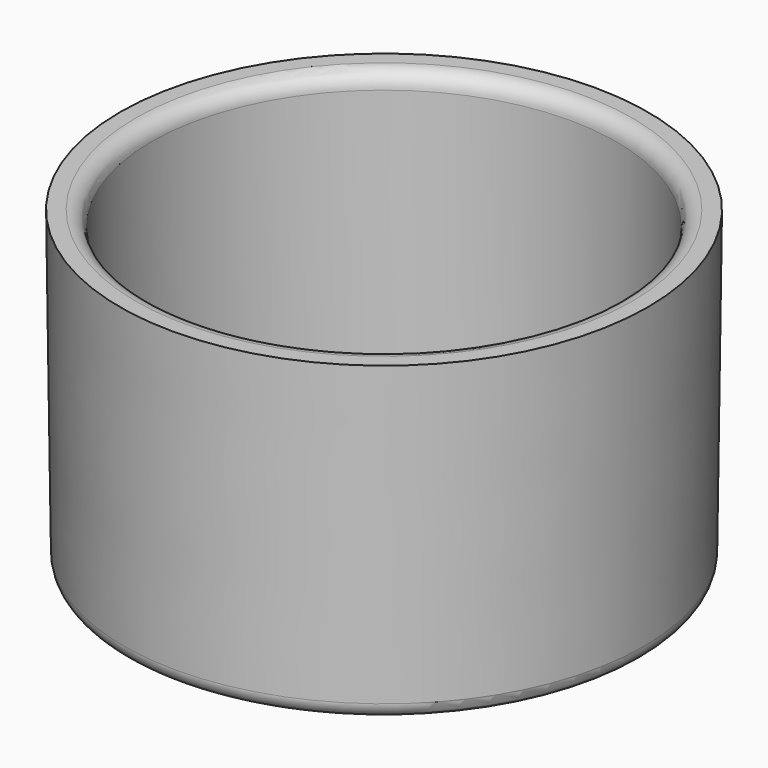
from build123d import *

# Parameters (mm, degrees)
F0_W     = 4
F0_H     = 40
F3_SIZE2 = 39.99999
F3_SIZE  = 0.49999
F4_R     = 2


# Not quite as in the source:
# - a fillet or chamfer is up to 0.001 mm smaller than in the source, because OpenCascade refuses the exact size


with BuildPart() as f2:
    # F0 (on Front) → F2 (revolve)
    with BuildSketch(Plane.XZ):
        with Locations((31.5, 20)):
            Rectangle(F0_W, F0_H)
    revolve(axis=Axis((0, 0, 14.9673912674), (0, 0, 1)))

    # F3 (size 0.5 and 40 in the source; OpenCascade refuses exactly that, so slightly less here)
    f3_edges = [f2.edges().sort_by_distance(p)[0] for p in [
        (-33.5, 0, 0),
    ]]
    chamfer(f3_edges, length=F3_SIZE, length2=F3_SIZE2)

    # F4
    f4_edges = [f2.edges().sort_by_distance(p)[0] for p in [
        (-29.5, 0, 40),
        (-33.00001, 0, 0),
    ]]
    fillet(f4_edges, radius=F4_R)


solid = f2.part
